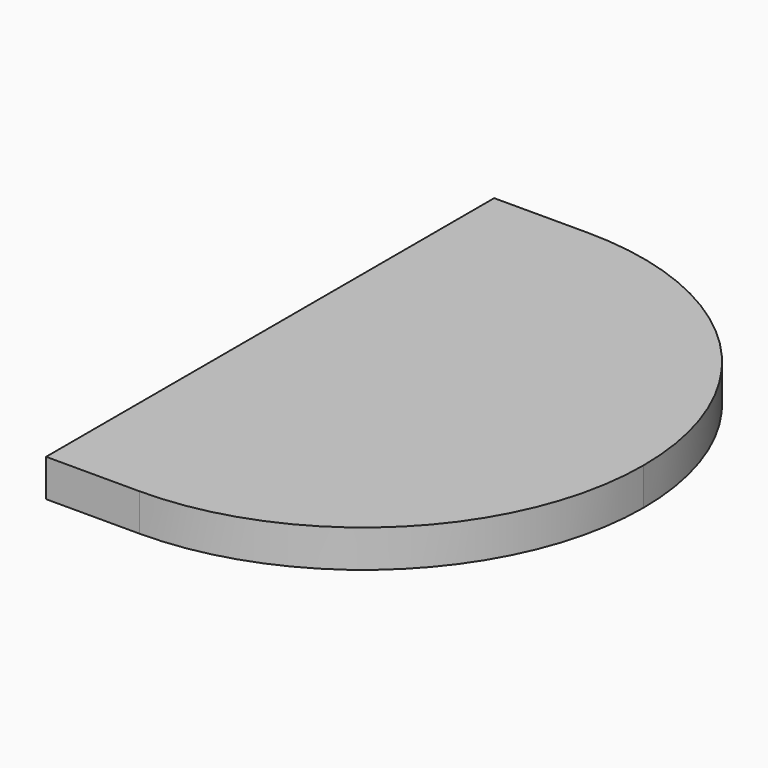
from build123d import *

# Parameters (mm, degrees)
F0_W     = 20
F0_H     = 30
F1_DEPTH = 2
F2_R     = 14.99999


# Not quite as in the source:
# - a fillet or chamfer is up to 0.001 mm smaller than in the source, because OpenCascade refuses the exact size


with BuildPart() as f1:
    # F0 (on Top) → F1 (new body)
    with BuildSketch(Plane.XY):
        with Locations((-9.3508988675, -20609.1883584166)):
            Rectangle(F0_W, F0_H)
    extrude(amount=F1_DEPTH)

    # F2 (radius 15 in the source; OpenCascade refuses exactly that, so slightly less here)
    f2_edges = [f1.edges().sort_by_distance(p)[0] for p in [
        (0.649101, -20594.188358, 1),
        (0.649101, -20624.188358, 1),
    ]]
    fillet(f2_edges, radius=F2_R)


solid = f1.part
